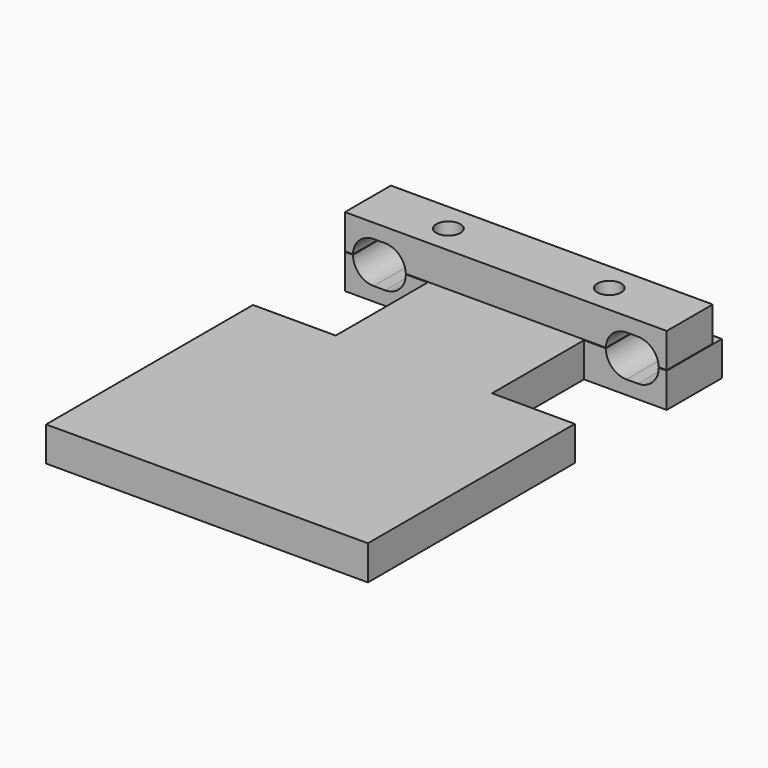
from build123d import *

# Parameters (mm, degrees)
F0_W      = 13.6
F0_H      = 6
F0_W_2    = 3.8
F1_DEPTH  = 12
F4_DEPTH  = 10
F3_R      = 2.1
F5_DEPTH  = 25
F3_R_2    = 2.5
F6_DEPTH  = 25
F8_DEPTH  = 65
F9_W      = 14.4
F9_H      = 45
F10_DEPTH = 6


# Not quite as in the source:
# - a feature of the source that left no trace in its solid (it failed there, or was rolled back) is left out


with BuildPart() as f1:
    # F0 (on Front) → F1 (new body)
    with BuildSketch(Plane.XZ):
        with Locations((6.8, -3)):
            Rectangle(F0_W, F0_H)
        with Locations((15.5, -3)):
            Rectangle(F0_W_2, F0_H)
        with Locations((-15.5, -3)):
            Rectangle(F0_W_2, F0_H)
        with Locations((-6.8, -3)):
            Rectangle(F0_W, F0_H)
        with BuildLine():
            Line((-17.4, -6), (-17.4, 0))
            ThreePointArc((-17.4, 0), (-18.4544155877, -2.5455844123), (-21, -3.6))
            Line((-21, -3.6), (-23, -3.6))
            ThreePointArc((-23, -3.6), (-25.5455844123, -2.5455844123), (-26.6, 0))
            Line((-26.6, 0), (-28, 0))
            Line((-28, 0), (-28, -6))
            Line((-28, -6), (-17.4, -6))
        make_face()
        with BuildLine():
            ThreePointArc((21, -3.6), (18.4544155877, -2.5455844123), (17.4, 0))
            Line((17.4, 0), (17.4, -6))
            Line((17.4, -6), (28, -6))
            Line((28, -6), (28, 0))
            Line((28, 0), (26.6, 0))
            ThreePointArc((26.6, 0), (25.5455844123, -2.5455844123), (23, -3.6))
            Line((23, -3.6), (21, -3.6))
        make_face()
    extrude(amount=-F1_DEPTH)

    # F3 (on Top) → F6 (cut)
    with BuildSketch(Plane.XY):
        with Locations((-14, 5)):
            Circle(F3_R_2)
        with Locations((-14, 5)):
            Circle(F3_R, mode=Mode.SUBTRACT)
        with Locations((14, 5)):
            Circle(F3_R_2)
        with Locations((14, 5)):
            Circle(F3_R, mode=Mode.SUBTRACT)
        with Locations((-14, 5)):
            Circle(F3_R)
        with Locations((14, 5)):
            Circle(F3_R)
    extrude(amount=-F6_DEPTH, mode=Mode.SUBTRACT)

    # F0 (on Front) → F8 (join)
    with BuildSketch(Plane.XZ):
        with Locations((-6.8, -3)):
            Rectangle(F0_W, F0_H)
        with Locations((6.8, -3)):
            Rectangle(F0_W, F0_H)
    extrude(amount=F8_DEPTH)

    # F9 (on face) → F10 (join)
    with BuildSketch(Plane.XY):
        with Locations((-20.8, -42.5)):
            Rectangle(F9_W, F9_H)
        with Locations((20.8, -42.5)):
            Rectangle(F9_W, F9_H)
    extrude(amount=-F10_DEPTH)


with BuildPart() as f4:
    # F0 (on Front) → F4 (new body)
    with BuildSketch(Plane.XZ):
        with BuildLine():
            Line((-17.4013891569, 0.1), (17.4013891569, 0.1))
            ThreePointArc((17.4013891569, 0.1), (18.4900199204, 2.5806975801), (21, 3.6))
            Line((21, 3.6), (23, 3.6))
            ThreePointArc((23, 3.6), (25.5099800796, 2.5806975801), (26.5986108431, 0.1))
            Line((26.5986108431, 0.1), (28, 0.1))
            Line((28, 0.1), (28, 6.1))
            Line((28, 6.1), (-28, 6.1))
            Line((-28, 6.1), (-28, 0.1))
            Line((-28, 0.1), (-26.5986108431, 0.1))
            ThreePointArc((-26.5986108431, 0.1), (-25.5099800796, 2.5806975801), (-23, 3.6))
            Line((-23, 3.6), (-21, 3.6))
            ThreePointArc((-21, 3.6), (-18.4900199204, 2.5806975801), (-17.4013891569, 0.1))
        make_face()
    extrude(amount=-F4_DEPTH)

    # F3 (on Top) → F5 (cut)
    with BuildSketch(Plane.XY):
        with Locations((14, 5)):
            Circle(F3_R)
        with Locations((-14, 5)):
            Circle(F3_R)
    extrude(amount=F5_DEPTH, mode=Mode.SUBTRACT)


solid = Compound([f1.part, f4.part])
